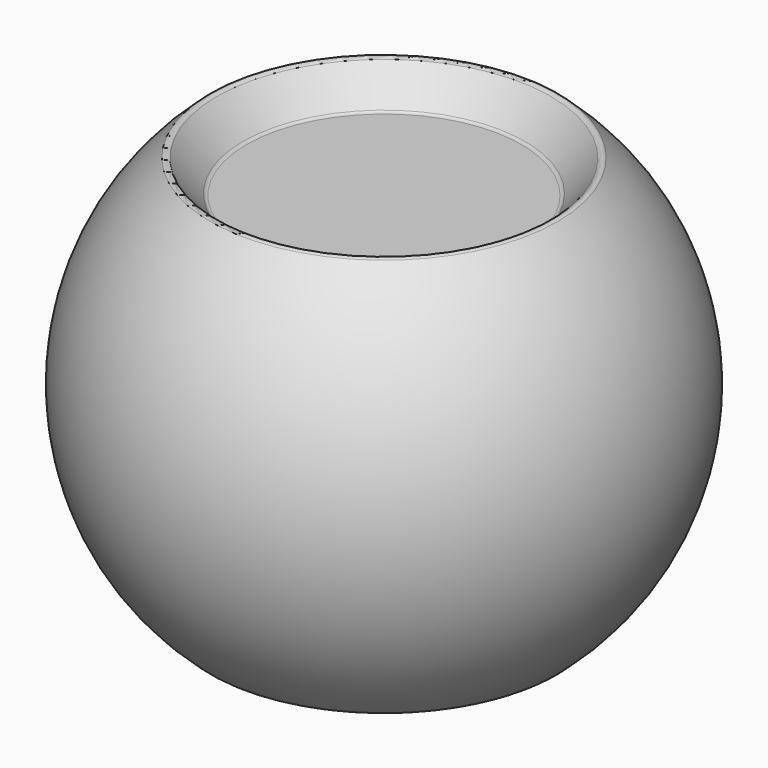
from build123d import *

# Parameters (mm, degrees)
F2_R = 0.5


with BuildPart() as f1:
    # F0 (on Front) → F1 (revolve)
    with BuildSketch(Plane.XZ):
        with BuildLine():
            ThreePointArc((-18.4254318222, 21.9076391525), (-18.7695123684, 22.084726587), (-19.1369191934, 21.963221004))
            ThreePointArc((-19.1369191934, 21.963221004), (-29.1307947208, -0.0393957284), (-19.0774443259, -22.0149011144))
            ThreePointArc((-19.0774443259, -22.0149011144), (-18.5423008943, -22.0918582573), (-18.25, -21.6370384232))
            Line((-18.25, -21.6370384232), (-18.25, -6.7055555556))
            Line((-18.25, -6.7055555556), (-7.9, -6.7055555556))
            Line((-7.9, -6.7055555556), (-7.9, -11.2055555556))
            Line((-7.9, -11.2055555556), (-5.15, -11.2055555556))
            Line((-5.15, -11.2055555556), (-5.15, -6.7055555556))
            Line((-5.15, -6.7055555556), (-5.15, 14.3005384632))
            Line((-5.15, 14.3005384632), (0, 14.3005384632))
            Line((0, 14.3005384632), (0, 18.3005384632))
            Line((0, 18.3005384632), (-15.3987149642, 18.3005384632))
            Line((-15.3987149642, 18.3005384632), (-18.4254318222, 21.9076391525))
        make_face()
    revolve(axis=Axis((0, 0, 1.3541673665), (0, 0, -1)))

    # F2
    f2_edges = [f1.edges().sort_by_distance(p)[0] for p in [
        (15.398715, 0, 18.300538),
        (18.25, 0, -6.705556),
        (5.15, 0, 14.300538),
    ]]
    fillet(f2_edges, radius=F2_R)


solid = f1.part
